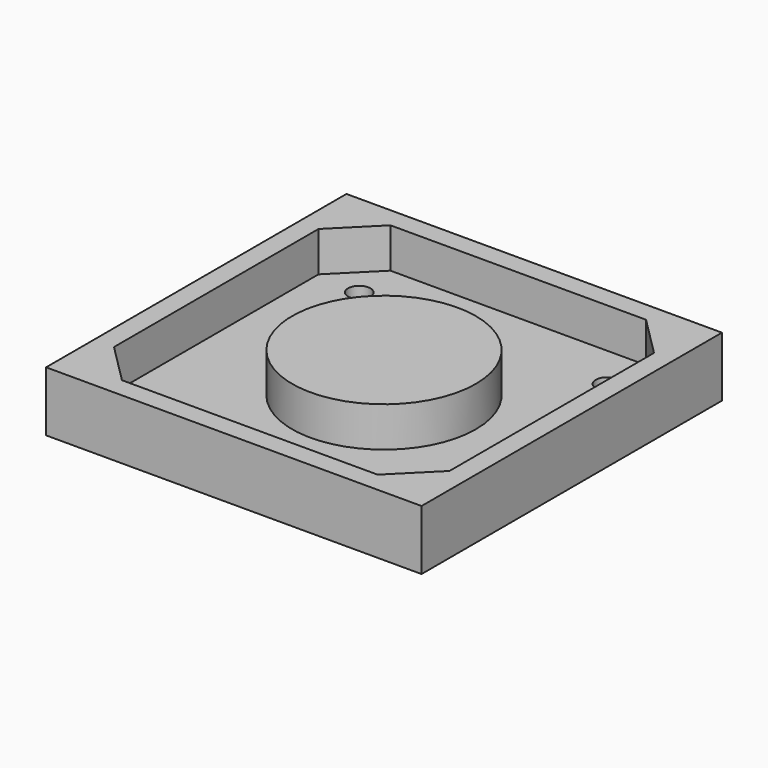
from build123d import *

# Parameters (mm, degrees)
F0_W        = 42
F0_H        = 42
F0_R        = 1.4
F0_R_2      = 11.5
F1_DEPTH    = 5
F2_T        = 2.5
F3_T1_DEPTH = 5
F4_DEPTH    = 5
F5_DEPTH    = 25


# Not quite as in the source:
# - a fillet or chamfer that OpenCascade refuses, or shapes differently, is made with other operations: its cross-section is extruded or revolved along the edge and cut away or added


with BuildPart() as f1:
    # F0 (on Top) → F1 (new body)
    with BuildSketch(Plane.XY):
        with Locations((-20.8238260887, 8.1392613277)):
            Rectangle(F0_W, F0_H)
        with Locations((-36.3238260887, -7.3607386723)):
            Circle(F0_R, mode=Mode.SUBTRACT)
        with Locations((-5.3238260887, -7.3607386723)):
            Circle(F0_R, mode=Mode.SUBTRACT)
        with Locations((-36.3238260887, 23.6392613277)):
            Circle(F0_R, mode=Mode.SUBTRACT)
        with Locations((-20.8238260887, 8.1392613277)):
            Circle(F0_R_2, mode=Mode.SUBTRACT)
        with Locations((-5.3238260887, 23.6392613277)):
            Circle(F0_R, mode=Mode.SUBTRACT)
        with Locations((-20.8238260887, 8.1392613277)):
            Circle(F0_R_2)
        with Locations((-36.3238260887, 23.6392613277)):
            Circle(F0_R)
        with Locations((-5.3238260887, 23.6392613277)):
            Circle(F0_R)
        with Locations((-5.3238260887, -7.3607386723)):
            Circle(F0_R)
        with Locations((-36.3238260887, -7.3607386723)):
            Circle(F0_R)
    extrude(amount=F1_DEPTH)

    # F2
    f2_openings = [f1.faces().sort_by_distance(p)[0] for p in [
        (-20.823826, 8.139261, 5),
    ]]
    offset(amount=F2_T, openings=f2_openings, kind=Kind.INTERSECTION)

    # F3: chamfer of 5 on 4 edges, made by hand

    # F3_s2 → F3_t1 (join)
    with BuildSketch(Plane.XY):
        Polygon((0.1761739113, -7.8607386723), (-4.8238260887, -12.8607386723), (0.1761739113, -12.8607386723), align=None)
        Polygon((0.1761739113, 24.1392613277), (-4.8238260887, 29.1392613277), (0.1761739113, 29.1392613277), align=None)
        Polygon((-36.8238260887, 29.1392613277), (-41.8238260887, 24.1392613277), (-41.8238260887, 29.1392613277), align=None)
        Polygon((-41.8238260887, -7.8607386723), (-36.8238260887, -12.8607386723), (-41.8238260887, -12.8607386723), align=None)
    extrude(amount=F3_T1_DEPTH)

    # F0 (on Top) → F4 (join)
    with BuildSketch(Plane.XY):
        with Locations((-20.8238260887, 8.1392613277)):
            Circle(F0_R_2)
    extrude(amount=F4_DEPTH)

    # F0 (on Top) → F5 (cut)
    with BuildSketch(Plane.XY):
        with Locations((-36.3238260887, -7.3607386723)):
            Circle(F0_R)
        with Locations((-36.3238260887, 23.6392613277)):
            Circle(F0_R)
        with Locations((-5.3238260887, 23.6392613277)):
            Circle(F0_R)
        with Locations((-5.3238260887, -7.3607386723)):
            Circle(F0_R)
    extrude(amount=-F5_DEPTH, mode=Mode.SUBTRACT)


solid = f1.part
